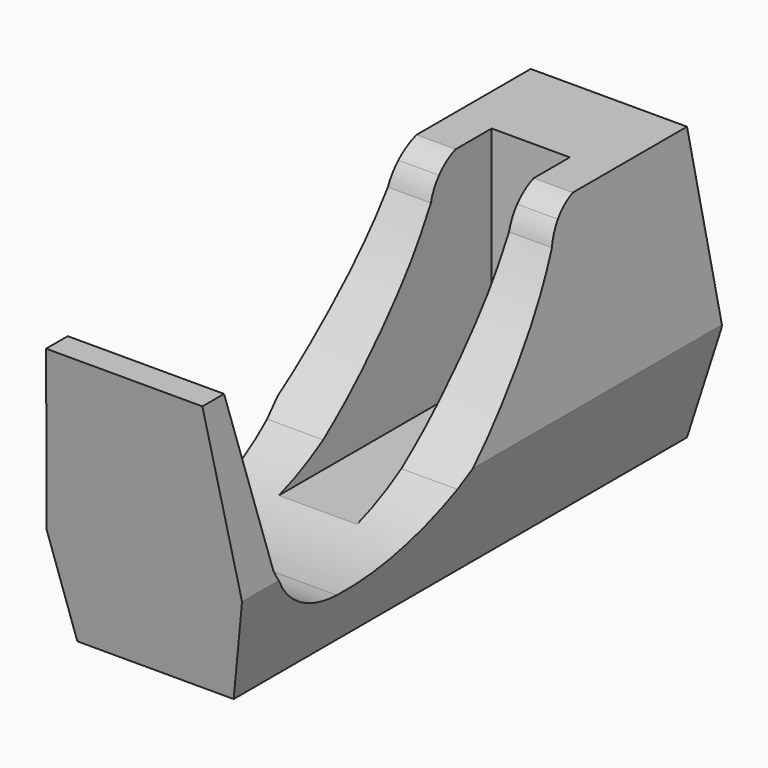
from build123d import *

# Parameters (mm, degrees)
F1_DEPTH = 160
F3_W     = 20
F3_H     = 75
F4_DEPTH = 55
F6_DEPTH = 80
F7_DEPTH = 80
F8_DEPTH = 200


with BuildPart() as f1:
    # F0 (on Front) → F1 (new body)
    with BuildSketch(Plane.XZ):
        Polygon((-21.2063081563, 25), (-16.2063081563, 70), (-21.2063081563, 70), align=None)
        Polygon((23.7936918437, 70), (-16.2063081563, 70), (-21.2063081563, 25), (-16.2063081563, 0), (23.7936918437, 0), (28.7936918437, 25), align=None)
        Polygon((28.7936918437, 70), (23.7936918437, 70), (28.7936918437, 25), align=None)
        Polygon((28.7936918437, 0), (28.7936918437, 25), (23.7936918437, 0), align=None)
        Polygon((-16.2063081563, 0), (-21.2063081563, 25), (-21.2063081563, 0), align=None)
    extrude(amount=F1_DEPTH)

    # F3 (on face) → F4 (cut)
    with BuildSketch(Plane.XY.offset(70)):
        with Locations((3.7936918437, -67.5)):
            Rectangle(F3_W, F3_H)
    extrude(amount=-F4_DEPTH, mode=Mode.SUBTRACT)

    # F5 (on face) → F6 (cut)
    with BuildSketch(Plane(origin=(-21.2063081563, 0, 0), x_dir=(0, -1, 0), z_dir=(-1, 0, 0))):
        with BuildLine():
            Line((120, 37), (120, 12))
            ThreePointArc((120, 12), (133.8212996215, 16.5538504991), (143.1985488392, 27.6818815335))
            Line((143.1985488392, 27.6818815335), (145.3737177065, 37))
            Line((145.3737177065, 37), (120, 37))
        make_face()
        with BuildLine():
            ThreePointArc((83.8675871491, 21.7687748373), (101.1727846043, 14.0695932653), (120, 12))
            Line((120, 12), (120, 37))
            Line((120, 37), (145.3737177065, 37))
            Line((145.3737177065, 37), (153.0770510435, 70))
            Line((153.0770510435, 70), (41.5276810527, 70))
            ThreePointArc((41.5276810527, 70), (44.4171997001, 68.4957364145), (46.8214808068, 66.2976555906))
            ThreePointArc((46.8214808068, 66.2976555906), (48.4316228068, 63.8555180083), (49.431870901, 61.1066824401))
            add(Edge.make_bspline(
                [(83.8675871491, 21.7687748373), (80.8791033045, 24.0777342993), (73.578379889, 29.6970945717), (57.4311562796, 47.0286131058), (51.4057960432, 57.3415797194), (49.431870901, 61.1066824401)],
                knots=[0, 0, 0, 0, 0.2722123221, 0.663175389, 0.8936579619, 0.8936579619, 0.8936579619, 0.8936579619], degree=3))
        make_face()
    extrude(amount=-F6_DEPTH, mode=Mode.SUBTRACT)

    # F2 (on face) → F7 (cut)
    with BuildSketch(Plane.YZ.offset(28.7936918437)):
        Polygon((-160, 0), (-150, 0), (-160, 70), (-160, 24.2114625871), align=None)
        Polygon((-5, 70), (0, 24.2114625871), (0, 70), align=None)
        Polygon((-5, 0), (0, 0), (0, 24.2114625871), align=None)
    extrude(amount=-F7_DEPTH, mode=Mode.SUBTRACT)

    # F0 (on Front) → F8 (cut)
    with BuildSketch(Plane.XZ):
        Polygon((28.7936918437, 70), (23.7936918437, 70), (28.7936918437, 25), align=None)
        Polygon((-21.2063081563, 25), (-16.2063081563, 70), (-21.2063081563, 70), align=None)
        Polygon((28.7936918437, 0), (28.7936918437, 25), (23.7936918437, 0), align=None)
        Polygon((-16.2063081563, 0), (-21.2063081563, 25), (-21.2063081563, 0), align=None)
    extrude(amount=F8_DEPTH, mode=Mode.SUBTRACT)


solid = f1.part
